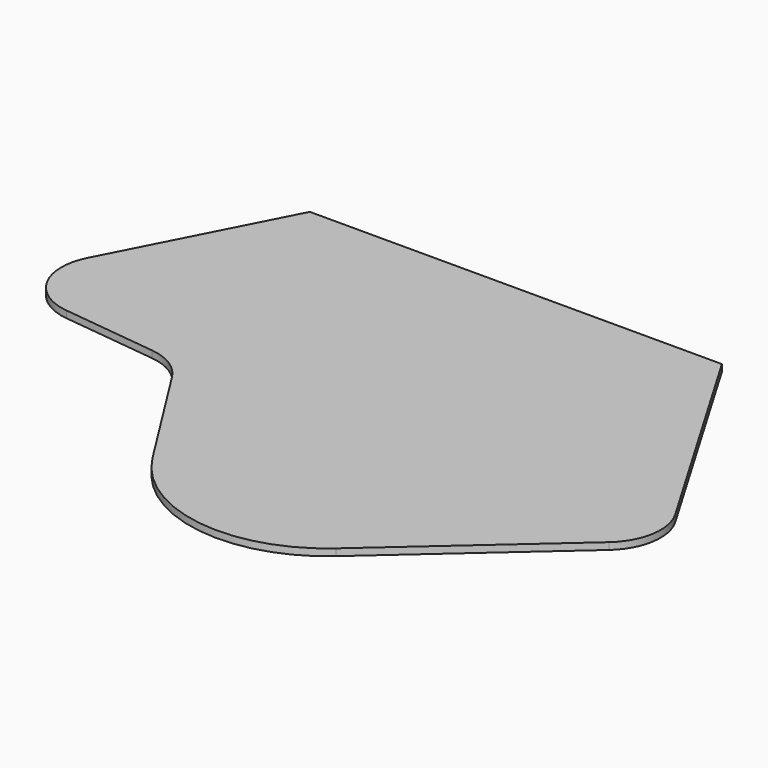
from build123d import *

# Parameters (mm, degrees)
F1_DEPTH = 1
F2_DEPTH = 25


# Not quite as in the source:
# - a feature names something its author has since deleted; it is built from what else it names


with BuildPart() as f1:
    # F0 (on Top) → F1 (new body)
    with BuildSketch(Plane.XY):
        with BuildLine():
            Line((9646.8274642131, -957.7307995355), (8146.8274642131, -957.7307995355))
            Line((8146.8274642131, -957.7307995355), (7830.554096613, -1573.7270701518))
            ThreePointArc((7830.554096613, -1573.7270701518), (7832.0390367178, -1759.2626053639), (7985.3704990637, -1863.7379734104))
            Line((7985.3704990637, -1863.7379734104), (8329.6804291381, -1903.7785528549))
            ThreePointArc((8329.6804291381, -1903.7785528549), (8413.0435068902, -1933.1322385833), (8475.616358081, -1995.5476204376))
            Line((8475.616358081, -1995.5476204376), (8744.9993562468, -2421.5486497246))
            ThreePointArc((8744.9993562468, -2421.5486497246), (9097.0590224145, -2649.3179001076), (9498.727349417, -2528.9543049258))
            Line((9498.727349417, -2528.9543049258), (10081.2209659321, -2014.102836222))
            ThreePointArc((10081.2209659321, -2014.102836222), (10146.2998029037, -1895.5752337571), (10121.0868255742, -1762.7281286256))
            Line((10121.0868255742, -1762.7281286256), (9646.8274642131, -957.7307995355))
        make_face()
    extrude(amount=F1_DEPTH)

    # F0 (on Top) → F2 (join)
    with BuildSketch(Plane.XY):
        with BuildLine():
            Line((9646.8274642131, -957.7307995355), (8146.8274642131, -957.7307995355))
            Line((8146.8274642131, -957.7307995355), (7830.554096613, -1573.7270701518))
            ThreePointArc((7830.554096613, -1573.7270701518), (7832.0390367178, -1759.2626053639), (7985.3704990637, -1863.7379734104))
            Line((7985.3704990637, -1863.7379734104), (8329.6804291381, -1903.7785528549))
            ThreePointArc((8329.6804291381, -1903.7785528549), (8413.0435068902, -1933.1322385833), (8475.616358081, -1995.5476204376))
            Line((8475.616358081, -1995.5476204376), (8744.9993562468, -2421.5486497246))
            ThreePointArc((8744.9993562468, -2421.5486497246), (9097.0590224145, -2649.3179001076), (9498.727349417, -2528.9543049258))
            Line((9498.727349417, -2528.9543049258), (10081.2209659321, -2014.102836222))
            ThreePointArc((10081.2209659321, -2014.102836222), (10146.2998029037, -1895.5752337571), (10121.0868255742, -1762.7281286256))
            Line((10121.0868255742, -1762.7281286256), (9646.8274642131, -957.7307995355))
        make_face()
    extrude(amount=F2_DEPTH)


solid = f1.part
